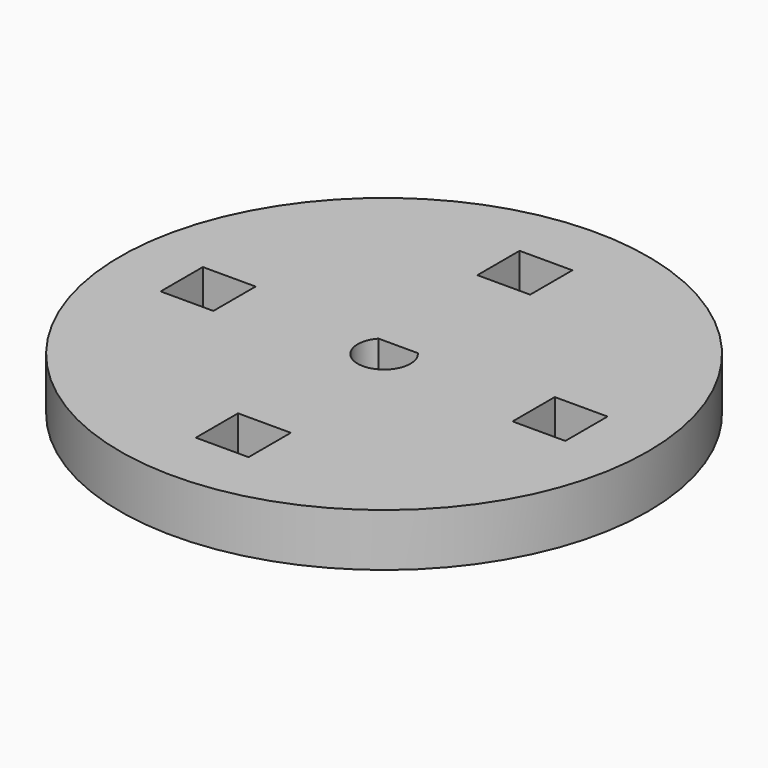
from build123d import *

# Parameters (mm, degrees)
F1_R            = 15
F2_DEPTH        = 3
F3_W            = 3
F3_H            = 3
F4_DEPTH        = 3
F4_COPIES_COUNT = 4
F6_DEPTH        = 3


# Not quite as in the source:
# - a pattern or mirror of a feature is missing from the dataset's text; its kind, count and spacing are read off the source's solid


with BuildPart() as f2:
    # F1 (on Top) → F2 (new body)
    with BuildSketch(Plane.XY):
        Circle(F1_R)
    extrude(amount=-F2_DEPTH)

    # F3 (on face) → F4 (cut, through all)
    with BuildSketch(Plane.XY):
        with Locations((-10, 0)):
            Rectangle(F3_W, F3_H)
    f4 = extrude(amount=-F4_DEPTH, mode=Mode.SUBTRACT)

    # F4_copies: F4 ×4 about axis
    f4_copies_axis = Axis((0, 0, 0), (0, 0, 1))
    for i in range(1, F4_COPIES_COUNT):
        add(f4.rotate(f4_copies_axis, i * 360 / F4_COPIES_COUNT), mode=Mode.SUBTRACT)

    # F5 (on face) → F6 (cut, through all)
    with BuildSketch(Plane.XY):
        with BuildLine():
            Line((1.1180339887, 1), (-1.1180339887, 1))
            ThreePointArc((-1.1180339887, 1), (0, -1.5), (1.1180339887, 1))
        make_face()
    extrude(amount=-F6_DEPTH, mode=Mode.SUBTRACT)


solid = f2.part
